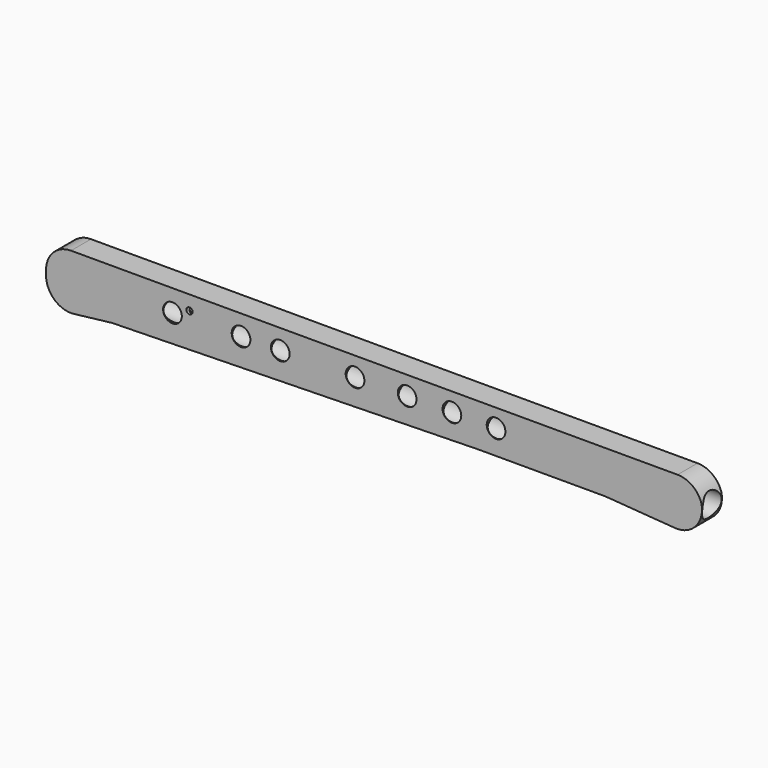
from build123d import *

# Parameters (mm, degrees)
F1_DEPTH    = 5.08
F2_R        = 1.905
F2_R_2      = 0.635
F3_DEPTH    = 5.081
F5_R        = 2.482268849
F6_DEPTH    = 135.1903097162
F7_T1_DEPTH = 30.48
F7_T3_DEPTH = 33.6434104505
F8_T1_DEPTH = 24.911720067
F8_T3_DEPTH = 40.2155938888


# Not quite as in the source:
# - a fillet or chamfer that OpenCascade refuses, or shapes differently, is made with other operations: its cross-section is extruded or revolved along the edge and cut away or added


with BuildPart() as f1:
    # F0 (on Front) → F1 (new body)
    with BuildSketch(Plane.XZ):
        Polygon((64.8356899619, 14.7801730782), (-67.7917227149, 14.7801730782), (-67.7917227149, 2.9560343828), (-54.3910339475, 4.5325863175), (20.2981028706, 6.1091380194), (46.1141429842, 6.1091380194), (67.3975870013, 4.5325863175), align=None)
    extrude(amount=F1_DEPTH)

    # F2 (on face) → F3 (cut, through all)
    with BuildSketch(Plane.XZ.offset(5.08)):
        with Locations((-42.0428626239, 10.3493910283)):
            Circle(F2_R)
        with Locations((-28.0725583434, 10.6500703841)):
            Circle(F2_R)
        with Locations((-20.0785025954, 10.7159726322)):
            Circle(F2_R)
        with Locations((5.7720425539, 10.9793273732)):
            Circle(F2_R)
        with Locations((-4.8454641365, 10.8956610784)):
            Circle(F2_R)
        with Locations((14.8922726512, 11.0351899639)):
            Circle(F2_R)
        with Locations((23.8888021559, 11.0784396529)):
            Circle(F2_R)
        with Locations((-38.571305573, 11.8272872642)):
            Circle(F2_R_2)
    extrude(amount=-F3_DEPTH, mode=Mode.SUBTRACT)

    # F5 (on face) → F6 (cut, through all)
    with BuildSketch(Plane(origin=(-67.7917227149, 0, 0), x_dir=(0, -1, 0), z_dir=(-1, 0, 0))):
        with Locations((2.5438587181, 9.8215453327)):
            Circle(F5_R)
    extrude(amount=-F6_DEPTH, mode=Mode.SUBTRACT)

    # F7: fillet of radius 5.08 on 2 edges, made by hand

    # F7_s2 → F7_t1 (cut)
    with BuildSketch(Plane.XZ.offset(-12.7)):
        with BuildLine():
            ThreePointArc((-67.7917227149, 9.7001730782), (-66.3038251633, 13.2922755266), (-62.7117227149, 14.7801730782))
            Line((-62.7117227149, 14.7801730782), (-67.7917227149, 14.7801730782))
            Line((-67.7917227149, 14.7801730782), (-67.7917227149, 9.7001730782))
        make_face()
    extrude(amount=F7_T1_DEPTH, mode=Mode.SUBTRACT)

    # F7_s4 → F7_t3 (cut)
    with BuildSketch(Plane.XZ.offset(-14.2817052253)):
        with BuildLine():
            ThreePointArc((-62.1181690603, 3.6235114167), (-66.0874557786, 4.8725570607), (-67.7917227149, 8.6687164729))
            Line((-67.7917227149, 8.6687164729), (-67.7917227149, 2.9560343828))
            Line((-67.7917227149, 2.9560343828), (-62.1181690603, 3.6235114167))
        make_face()
    extrude(amount=F7_T3_DEPTH, mode=Mode.SUBTRACT)

    # F8: fillet of radius 5.08 on 2 edges, made by hand

    # F8_s2 → F8_t1 (cut)
    with BuildSketch(Plane.XZ.offset(-9.9158600335)):
        with BuildLine():
            ThreePointArc((65.7976698097, 10.9322542114), (63.9956399081, 13.7042567534), (60.8693459485, 14.7801730782))
            Line((60.8693459485, 14.7801730782), (64.8356899619, 14.7801730782))
            Line((64.8356899619, 14.7801730782), (65.7976698097, 10.9322542114))
        make_face()
    extrude(amount=F8_T1_DEPTH, mode=Mode.SUBTRACT)

    # F8_s4 → F8_t3 (cut)
    with BuildSketch(Plane.XZ.offset(-17.5677969444)):
        with BuildLine():
            ThreePointArc((60.3896680446, 5.051691522), (64.6507327019, 6.8456585743), (65.6932601377, 11.3498928427))
            Line((65.6932601377, 11.3498928427), (67.3975870013, 4.5325863175))
            Line((67.3975870013, 4.5325863175), (60.3896680446, 5.051691522))
        make_face()
    extrude(amount=F8_T3_DEPTH, mode=Mode.SUBTRACT)


solid = f1.part
